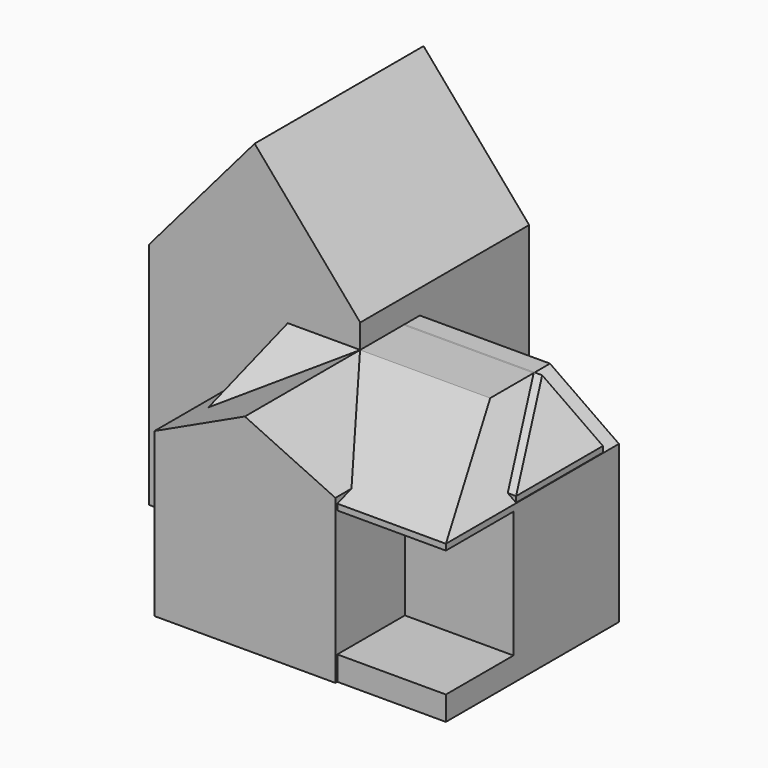
from build123d import *

# Parameters (mm, degrees)
F1_DEPTH  = 3895
F2_W      = 2145
F2_H      = 1200
F2_W_2    = 120
F3_REACH  = 5862.8506699351
F6_DEPTH  = 3500
F7_W      = 780
F7_H      = 1200
F8_DEPTH  = 50
F10_DEPTH = 2190
F13_DEPTH = 3600
F16_DEPTH = 4500
F18_DEPTH = 4050
F19_W     = 2200
F19_H     = 2100
F20_DEPTH = 1400


with BuildPart() as f1:
    # F0 (on Right) → F1 (new body)
    with BuildSketch(Plane.YZ):
        Polygon((-1200, 0), (0, 0), (0, 2700), (-1200, 2230), align=None)
        Polygon((0, 2700), (0, 0), (1800, 0), (1800, 3405), align=None)
    extrude(amount=F1_DEPTH)

    f3_end = f1.faces().sort_by_distance((1947.5, 300, 2817.5))[0]
    # F2 (on Top) → F3 (cut, up to a face of the model that its end follows)
    with BuildSketch(Plane.XY):
        with Locations((2822.5, -600)):
            Rectangle(F2_W, F2_H)
        with Locations((60, -600)):
            Rectangle(F2_W_2, F2_H)
    f3_long = extrude(amount=F3_REACH, mode=Mode.PRIVATE)
    add(split(f3_long, bisect_by=f3_end, keep=Keep.BOTTOM, mode=Mode.PRIVATE), mode=Mode.SUBTRACT)

    # F5 (on offset) → F6 (join)
    with BuildSketch(Plane.XZ.offset(-890)):
        Polygon((-2900, 0), (600, 0), (600, 3800), (-1150, 5841.6666666667), (-2900, 3800), align=None)
    extrude(amount=-F6_DEPTH)

    # F7 (on face) → F8 (cut)
    with BuildSketch(Plane.XZ):
        with Locations((2655, 1700)):
            Rectangle(F7_W, F7_H)
    extrude(amount=-F8_DEPTH, mode=Mode.SUBTRACT)

    # F9 (on face) → F10 (cut)
    with BuildSketch(Plane.XZ):
        Polygon((2888.1556552468, 3405), (3895, 2700), (3895, 3405), align=None)
    extrude(amount=-F10_DEPTH, mode=Mode.SUBTRACT)


with BuildPart() as f13:
    # F12 (on offset) → F13 (new body)
    with BuildSketch(Plane.XZ.offset(1500)):
        Polygon((2100, 2700), (600, 3400), (-900, 2700), (-900, 0), (600, 0), (2100, 0), align=None)
    extrude(amount=-F13_DEPTH)


with BuildPart() as f16:
    # F15 (on offset) → F16 (new body)
    with BuildSketch(Plane.YZ.offset(-600)):
        Polygon((2125.2750161739, 3400), (886.8726551098, 3400), (-1460, 2600), (-1460, 0), (2125.2750161739, 0), align=None)
    extrude(amount=F16_DEPTH)

    # F17 (on face) → F18 (cut)
    with BuildSketch(Plane.XZ.offset(1460)):
        Polygon((2757.4815946063, 3400), (3900, 2600), (3900, 3400), align=None)
    extrude(amount=-F18_DEPTH, mode=Mode.SUBTRACT)

    # F19 (on face) → F20 (cut)
    with BuildSketch(Plane.XZ.offset(1460)):
        with Locations((2800, 1450)):
            Rectangle(F19_W, F19_H)
    extrude(amount=-F20_DEPTH, mode=Mode.SUBTRACT)


solid = Compound([f1.part, f13.part, f16.part])
